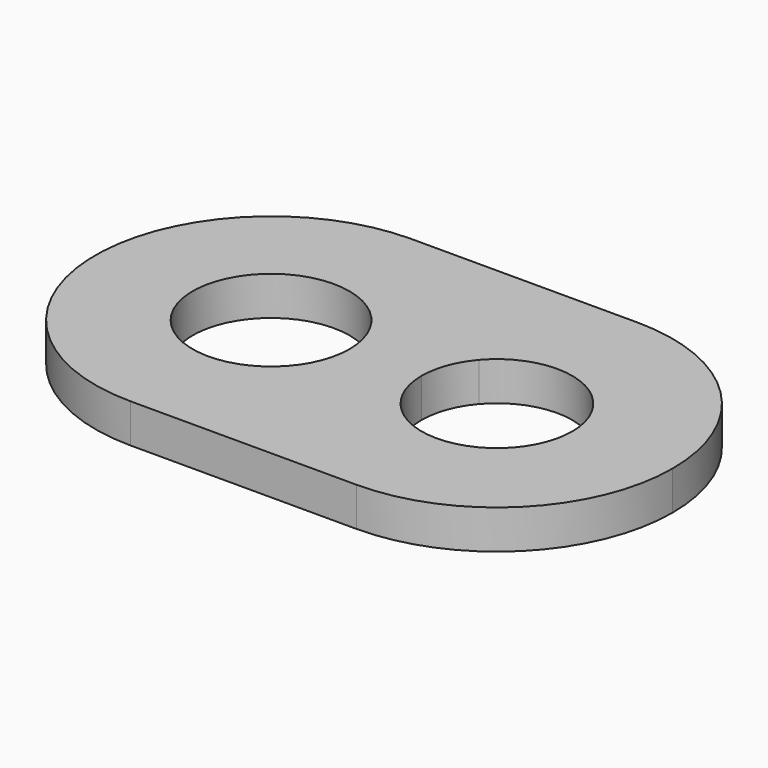
from build123d import *

# Parameters (mm, degrees)
F1_DEPTH = 3.1
F2_DEPTH = 3.1


# Not quite as in the source:
# - a feature names something its author has since deleted; it is built from what else it names


with BuildPart() as f1:
    # F0 (on Top) → F1 (new body)
    with BuildSketch(Plane.XY):
        with BuildLine():
            ThreePointArc((-38.8921249823, 64.9047296424), (-32.2549034273, 66.6273143387), (-28.3365694268, 61))
            ThreePointArc((-28.3365694268, 61), (-32.2549034273, 55.3726856613), (-38.8921249823, 57.0952703576))
            ThreePointArc((-38.8921249823, 57.0952703576), (-40.607834636, 53.3556046539), (-43.3365694268, 50.2761947052))
            ThreePointArc((-43.3365694268, 50.2761947052), (-39.1254485166, 47.8445206449), (-34.3365694268, 47))
            ThreePointArc((-34.3365694268, 47), (-24.4370744902, 51.1005050634), (-20.3365694268, 61))
            ThreePointArc((-20.3365694268, 61), (-24.4370744902, 70.8994949366), (-34.3365694268, 75))
            ThreePointArc((-34.3365694268, 75), (-39.1254485166, 74.1554793551), (-43.3365694268, 71.7238052948))
            ThreePointArc((-43.3365694268, 71.7238052948), (-40.607834636, 68.6443953461), (-38.8921249823, 64.9047296424))
        make_face()
        with BuildLine():
            ThreePointArc((-52.3365694268, 75), (-47.547690337, 74.1554793551), (-43.3365694268, 71.7238052948))
            ThreePointArc((-43.3365694268, 71.7238052948), (-39.1254485166, 74.1554793551), (-34.3365694268, 75))
            Line((-34.3365694268, 75), (-52.3365694268, 75))
        make_face()
        with BuildLine():
            ThreePointArc((-47.6959444268, 65.1865379025), (-45.9842893254, 68.7672788776), (-43.3365694268, 71.7238052948))
            ThreePointArc((-43.3365694268, 71.7238052948), (-47.547690337, 74.1554793551), (-52.3365694268, 75))
            ThreePointArc((-52.3365694268, 75), (-66.3365694268, 61), (-52.3365694268, 47))
            ThreePointArc((-52.3365694268, 47), (-47.547690337, 47.8445206449), (-43.3365694268, 50.2761947052))
            ThreePointArc((-43.3365694268, 50.2761947052), (-45.9842893254, 53.2327211224), (-47.6959444268, 56.8134620975))
            ThreePointArc((-47.6959444268, 56.8134620975), (-58.5865694268, 61), (-47.6959444268, 65.1865379025))
        make_face()
        with BuildLine():
            ThreePointArc((-34.3365694268, 47), (-39.1254485166, 47.8445206449), (-43.3365694268, 50.2761947052))
            ThreePointArc((-43.3365694268, 50.2761947052), (-47.547690337, 47.8445206449), (-52.3365694268, 47))
            Line((-52.3365694268, 47), (-34.3365694268, 47))
        make_face()
        with BuildLine():
            ThreePointArc((-40.3365694268, 61), (-39.9638837655, 63.0816659995), (-38.8921249823, 64.9047296424))
            ThreePointArc((-38.8921249823, 64.9047296424), (-40.607834636, 68.6443953461), (-43.3365694268, 71.7238052948))
            ThreePointArc((-43.3365694268, 71.7238052948), (-45.9842893254, 68.7672788776), (-47.6959444268, 65.1865379025))
            ThreePointArc((-47.6959444268, 65.1865379025), (-46.5027710822, 63.2426093898), (-46.0865694268, 61))
            Line((-46.0865694268, 61), (-40.3365694268, 61))
        make_face()
        with BuildLine():
            ThreePointArc((-43.3365694268, 50.2761947052), (-40.607834636, 53.3556046539), (-38.8921249823, 57.0952703576))
            ThreePointArc((-38.8921249823, 57.0952703576), (-39.9638837655, 58.9183340005), (-40.3365694268, 61))
            Line((-40.3365694268, 61), (-46.0865694268, 61))
            ThreePointArc((-46.0865694268, 61), (-46.5027710822, 58.7573906102), (-47.6959444268, 56.8134620975))
            ThreePointArc((-47.6959444268, 56.8134620975), (-45.9842893254, 53.2327211224), (-43.3365694268, 50.2761947052))
        make_face()
    extrude(amount=F1_DEPTH)

    # F0 (on Top) → F2 (join)
    with BuildSketch(Plane.XY):
        with BuildLine():
            ThreePointArc((-38.8921249823, 64.9047296424), (-32.2549034273, 66.6273143387), (-28.3365694268, 61))
            ThreePointArc((-28.3365694268, 61), (-32.2549034273, 55.3726856613), (-38.8921249823, 57.0952703576))
            ThreePointArc((-38.8921249823, 57.0952703576), (-40.607834636, 53.3556046539), (-43.3365694268, 50.2761947052))
            ThreePointArc((-43.3365694268, 50.2761947052), (-39.1254485166, 47.8445206449), (-34.3365694268, 47))
            ThreePointArc((-34.3365694268, 47), (-24.4370744902, 51.1005050634), (-20.3365694268, 61))
            ThreePointArc((-20.3365694268, 61), (-24.4370744902, 70.8994949366), (-34.3365694268, 75))
            ThreePointArc((-34.3365694268, 75), (-39.1254485166, 74.1554793551), (-43.3365694268, 71.7238052948))
            ThreePointArc((-43.3365694268, 71.7238052948), (-40.607834636, 68.6443953461), (-38.8921249823, 64.9047296424))
        make_face()
        with BuildLine():
            ThreePointArc((-52.3365694268, 75), (-47.547690337, 74.1554793551), (-43.3365694268, 71.7238052948))
            ThreePointArc((-43.3365694268, 71.7238052948), (-39.1254485166, 74.1554793551), (-34.3365694268, 75))
            Line((-34.3365694268, 75), (-52.3365694268, 75))
        make_face()
        with BuildLine():
            ThreePointArc((-47.6959444268, 65.1865379025), (-45.9842893254, 68.7672788776), (-43.3365694268, 71.7238052948))
            ThreePointArc((-43.3365694268, 71.7238052948), (-47.547690337, 74.1554793551), (-52.3365694268, 75))
            ThreePointArc((-52.3365694268, 75), (-66.3365694268, 61), (-52.3365694268, 47))
            ThreePointArc((-52.3365694268, 47), (-47.547690337, 47.8445206449), (-43.3365694268, 50.2761947052))
            ThreePointArc((-43.3365694268, 50.2761947052), (-45.9842893254, 53.2327211224), (-47.6959444268, 56.8134620975))
            ThreePointArc((-47.6959444268, 56.8134620975), (-58.5865694268, 61), (-47.6959444268, 65.1865379025))
        make_face()
        with BuildLine():
            ThreePointArc((-34.3365694268, 47), (-39.1254485166, 47.8445206449), (-43.3365694268, 50.2761947052))
            ThreePointArc((-43.3365694268, 50.2761947052), (-47.547690337, 47.8445206449), (-52.3365694268, 47))
            Line((-52.3365694268, 47), (-34.3365694268, 47))
        make_face()
    extrude(amount=F2_DEPTH)


solid = f1.part
